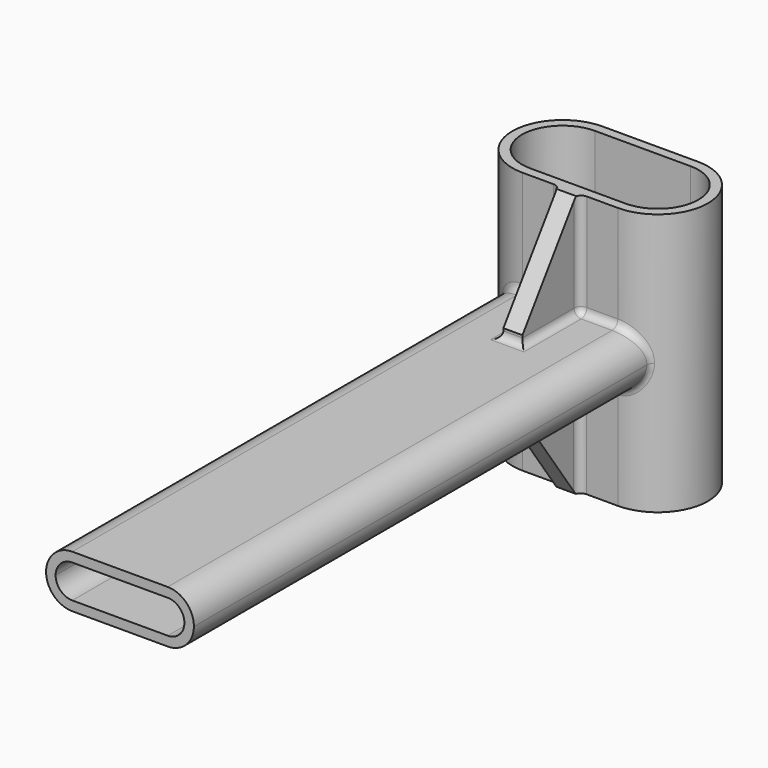
from build123d import *

# Parameters (mm, degrees)
F1_DEPTH = 27.5
F2_W     = 20
F2_H     = 2
F3_DEPTH = 120
F4_W     = 4
F4_H     = 22
F5_DEPTH = 15
F6_SIZE2 = 14.0041507642
F6_SIZE  = 20
F8_DEPTH = 15
F9_SIZE2 = 20
F9_SIZE  = 14.0041507642
F10_F1_R = 1.5
F10_F2_R = 1.5
F10_F3_R = 1.5
F10_F4_R = 1.5
F10_F5_R = 1.5
F10_F6_R = 1.5
F10_F7_R = 1.5
F10_F8_R = 1.5


# Not quite as in the source:
# - a feature names something its author has since deleted; it is built from what else it names


with BuildPart() as f1:
    # F0 (on Top) → F1 (new body, symmetric)
    with BuildSketch(Plane.XY):
        with BuildLine():
            Line((-10, -15.9872266478), (0, -15.9872266478))
            Line((0, -15.9872266478), (10, -15.9872266478))
            ThreePointArc((10, -15.9872266478), (20.5, -5.4872266478), (10, 5.0127733522))
            Line((10, 5.0127733522), (0, 5.0127733522))
            Line((0, 5.0127733522), (-10, 5.0127733522))
            ThreePointArc((-10, 5.0127733522), (-20.5, -5.4872266478), (-10, -15.9872266478))
        make_face()
        with BuildLine():
            Line((0, 3.0127733522), (10, 3.0127733522))
            ThreePointArc((10, 3.0127733522), (18.5, -5.4872266478), (10, -13.9872266478))
            Line((10, -13.9872266478), (0, -13.9872266478))
            Line((0, -13.9872266478), (-10, -13.9872266478))
            ThreePointArc((-10, -13.9872266478), (-18.5, -5.4872266478), (-10, 3.0127733522))
            Line((-10, 3.0127733522), (0, 3.0127733522))
        make_face(mode=Mode.SUBTRACT)
    extrude(amount=F1_DEPTH, both=True)

    # F2 (on face) → F3 (join)
    with BuildSketch(Plane(origin=(0, -13.9872266478, 0), x_dir=(-1, 0, 0), z_dir=(0, 1, 0))):
        with Locations((0, -4.5)):
            Rectangle(F2_W, F2_H)
        with BuildLine():
            ThreePointArc((-15.5, 0), (-13.8890872965, -3.8890872965), (-10, -5.5))
            Line((-10, -5.5), (-10, -3.5))
            ThreePointArc((-10, -3.5), (-12.4748737342, -2.4748737342), (-13.5, 0))
            ThreePointArc((-13.5, 0), (-12.4748737342, 2.4748737342), (-10, 3.5))
            Line((-10, 3.5), (-10, 5.5))
            ThreePointArc((-10, 5.5), (-13.8890872965, 3.8890872965), (-15.5, 0))
        make_face()
        with BuildLine():
            Line((10, -3.5), (10, -5.5))
            ThreePointArc((10, -5.5), (13.8890872965, -3.8890872965), (15.5, 0))
            ThreePointArc((15.5, 0), (13.8890872965, 3.8890872965), (10, 5.5))
            Line((10, 5.5), (10, 3.5))
            ThreePointArc((10, 3.5), (12.4748737342, 2.4748737342), (13.5, 0))
            ThreePointArc((13.5, 0), (12.4748737342, -2.4748737342), (10, -3.5))
        make_face()
        with Locations((0, 4.5)):
            Rectangle(F2_W, F2_H)
    extrude(amount=-F3_DEPTH)

    # F4 (on face) → F5 (join)
    with BuildSketch(Plane.XZ.offset(15.9872266478)):
        with Locations((0, 16.5)):
            Rectangle(F4_W, F4_H)
    extrude(amount=F5_DEPTH)

    # F6
    f6_edges = [f1.edges().sort_by_distance(p)[0] for p in [
        (0, -30.987227, 27.5),
    ]]
    f6_side = f1.faces().sort_by_distance((0, -30.987227, 16.5))[0]
    chamfer(f6_edges, length=F6_SIZE, length2=F6_SIZE2, reference=f6_side)

    # F7 (on face) → F8 (join)
    with BuildSketch(Plane.XZ.offset(15.9872266478)):
        Polygon((1.9211450554, -5.5), (0, -5.5), (-2.0788549446, -5.5), (-2.0788549446, -27.5), (1.9211450554, -27.5), align=None)
    extrude(amount=F8_DEPTH)

    # F9
    f9_edges = [f1.edges().sort_by_distance(p)[0] for p in [
        (-0.078855, -30.987227, -27.5),
    ]]
    f9_side = f1.faces().sort_by_distance((-6.039427, -15.441608, -27.5))[0]
    chamfer(f9_edges, length=F9_SIZE, length2=F9_SIZE2, reference=f9_side)

    # F10: fillet of radius 1.5 on 12 edges, made by hand

    # F10_f1
    f10_f1_edges = [f1.edges().sort_by_distance(p)[0] for p in [
        (-2.0788549446, -15.9872266478, -16.5),
    ]]
    fillet(f10_f1_edges, radius=F10_F1_R)

    # F10_f2
    f10_f2_edges = [f1.edges().sort_by_distance(p)[0] for p in [
        (-2.0788549446, -24.2372266478, -5.5),
    ]]
    fillet(f10_f2_edges, radius=F10_F2_R)

    # F10_f3
    f10_f3_edges = [f1.edges().sort_by_distance(p)[0] for p in [
        (1.9211450554, -15.9872266478, -16.5),
    ]]
    fillet(f10_f3_edges, radius=F10_F3_R)

    # F10_f4
    f10_f4_edges = [f1.edges().sort_by_distance(p)[0] for p in [
        (1.9211450554, -24.2372266478, -5.5),
    ]]
    fillet(f10_f4_edges, radius=F10_F4_R)

    # F10_f5
    f10_f5_edges = [f1.edges().sort_by_distance(p)[0] for p in [
        (-0.0788549446, -30.9872266478, -5.5),
    ]]
    fillet(f10_f5_edges, radius=F10_F5_R)

    # F10_f6
    f10_f6_edges = [f1.edges().sort_by_distance(p)[0] for p in [
        (-2, -15.9872266478, 17.25),
    ]]
    fillet(f10_f6_edges, radius=F10_F6_R)

    # F10_f7
    f10_f7_edges = [f1.edges().sort_by_distance(p)[0] for p in [
        (2, -15.9872266478, 17.25),
    ]]
    fillet(f10_f7_edges, radius=F10_F7_R)

    # F10_f8
    f10_f8_edges = [f1.edges().sort_by_distance(p)[0] for p in [
        (0, -30.9872266478, 5.5),
    ]]
    fillet(f10_f8_edges, radius=F10_F8_R)


solid = f1.part
